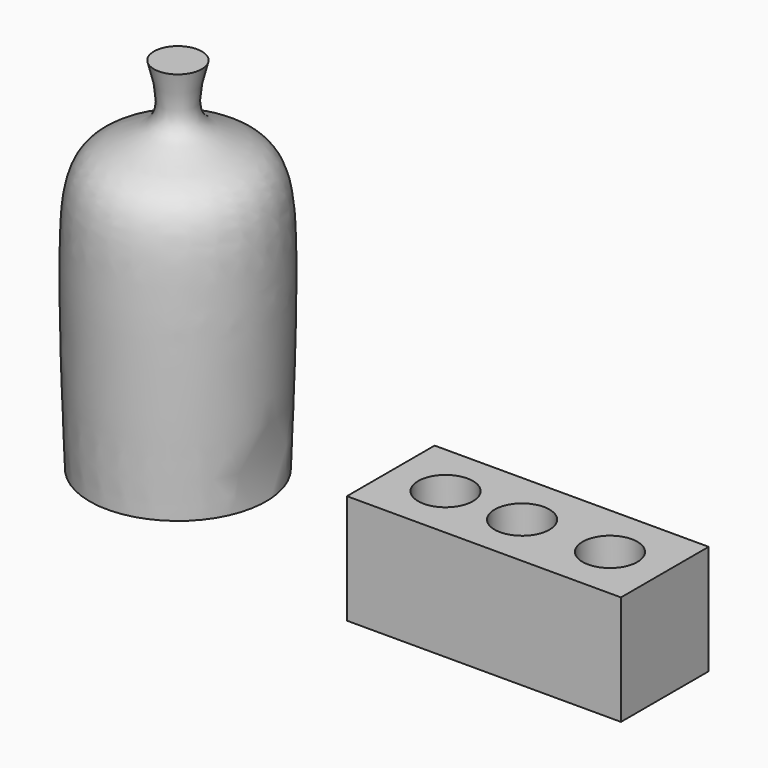
from build123d import *

# Parameters (mm, degrees)
F5_W     = 63.5
F5_H     = 25.4
F6_DEPTH = 25.4
F7_R     = 6.35
F8_DEPTH = 12.7


# Not quite as in the source:
# - a feature of the source that left no trace in its solid (it failed there, or was rolled back) is left out


with BuildPart() as f4:
    # F3 (on Front) → F4 (revolve)
    with BuildSketch(Plane.XZ):
        with BuildLine():
            Line((-46.2280027568, 31.3372500241), (-51.7842508852, 31.3372500241))
            add(Edge.make_bspline(
                [(-51.7842508852, 31.3372500241), (-50.5211565441, 26.7471574214), (-47.9211324049, 17.2986537112), (-66.2013951665, 14.212463315), (-68.335106942, -6.0060096659), (-67.3143122563, -34.2915675348), (-66.6749998927, -52.0064979792)],
                knots=[0, 0, 0, 0, 0.1904381048, 0.3920084616, 0.6192216585, 1, 1, 1, 1], degree=3))
            add(Edge.make_bspline(
                [(-66.6749998927, -52.0064979792), (-59.8593341808, -52.0064979792), (-53.0436684688, -52.0064979792), (-46.2280027568, -52.0064979792)],
                knots=[0, 0, 0, 0, 20.4469971359, 20.4469971359, 20.4469971359, 20.4469971359], degree=3))
            Line((-46.2280027568, -52.0064979792), (-46.2280027568, 31.3372500241))
        make_face()
    revolve(axis=Axis((-46.2280027568, 0, -10.3346239775), (0, 0, 1)))


with BuildPart() as f6:
    # F5 (on Front) → F6 (new body)
    with BuildSketch(Plane.XZ):
        with Locations((45.0056269765, -40.6170164633)):
            Rectangle(F5_W, F5_H)
    extrude(amount=F6_DEPTH)

    # F7 (on face) → F8 (cut)
    with BuildSketch(Plane.XY.offset(-27.9170164633)):
        with Locations((25.9556269765, -12.7)):
            Circle(F7_R)
        with Locations((43.7356269765, -12.7636595487)):
            Circle(F7_R)
        with Locations((64.0556269765, -12.7)):
            Circle(F7_R)
    extrude(amount=-F8_DEPTH, mode=Mode.SUBTRACT)


solid = Compound([f4.part, f6.part])
